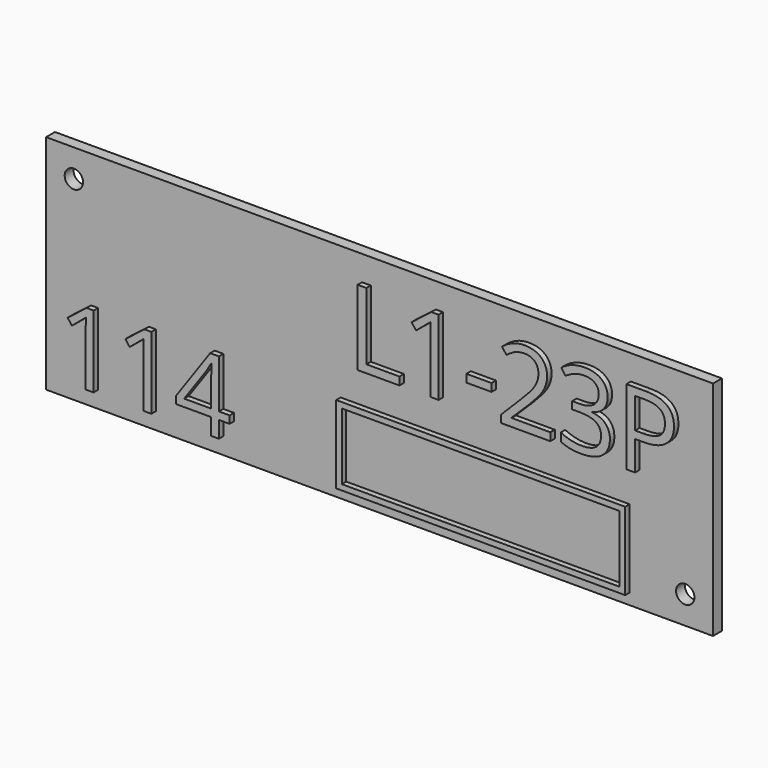
from build123d import *

# Parameters (mm, degrees)
F0_W         = 120
F0_H         = 40
F1_DEPTH     = 2
F3_D         = 3.3
F4_TEXT_SIZE = 18.9181200118
F5_DEPTH     = 1
F6_TEXT_SIZE = 18.1818181818
F7_DEPTH     = 1
F8_W         = 52
F8_H         = 14
F8_W_2       = 49.99999962
F8_H_2       = 11.99999962
F9_DEPTH     = 1


# Not quite as in the source:
# - Text() gives the source's letters only with a copy of the font that has no kerning and outlines rounded to 1/6400 em; it was checked with that copy


with BuildPart() as f1:
    # F0 (on Front) → F1 (new body)
    with BuildSketch(Plane.XZ):
        Rectangle(F0_W, F0_H)
    extrude(amount=F1_DEPTH)

    # F3 (through all)
    with Locations(Plane.XZ.offset(2)):
        with Locations((-55, 15), (55, -15)):
            Hole(F3_D / 2)

    # F4 (on face) → F5 (join)
    with BuildSketch(Plane.XZ.offset(2)):
        with Locations((-5, 2)):
            Text('L1-23P', F4_TEXT_SIZE, font='Open Sans', text_align=(TextAlign.LEFT, TextAlign.BOTTOM))
    extrude(amount=F5_DEPTH)

    # F6 (on face) → F7 (join)
    with BuildSketch(Plane.XZ.offset(2)):
        with Locations((-57, -17)):
            Text('114', F6_TEXT_SIZE, font='Open Sans', text_align=(TextAlign.LEFT, TextAlign.BOTTOM))
    extrude(amount=F7_DEPTH)

    # F8 (on face) → F9 (join)
    with BuildSketch(Plane.XZ.offset(2)):
        with Locations((19, -11)):
            Rectangle(F8_W, F8_H)
        with Locations((19, -11)):
            Rectangle(F8_W_2, F8_H_2, mode=Mode.SUBTRACT)
    extrude(amount=F9_DEPTH)


solid = f1.part
